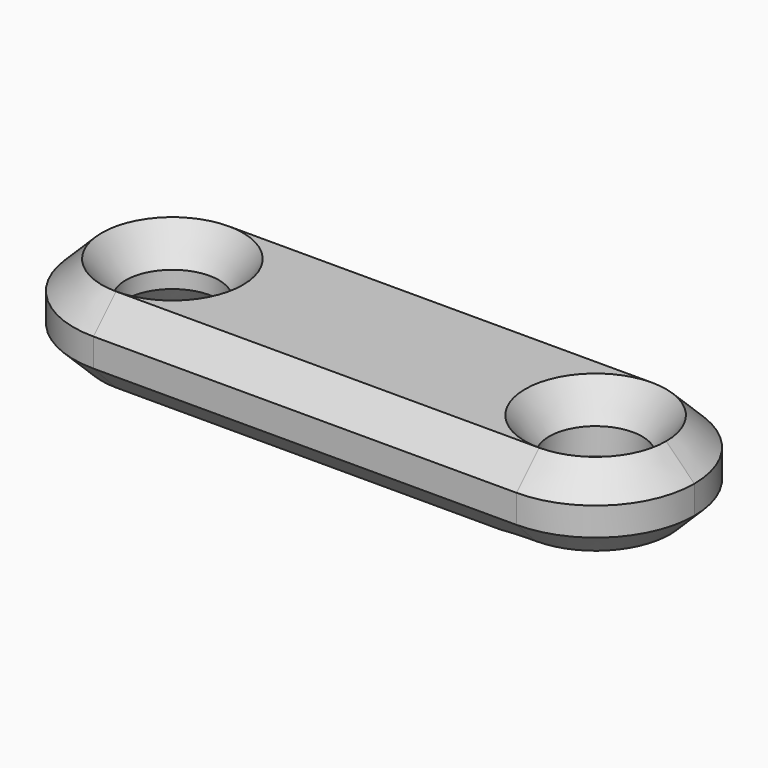
from build123d import *

# Parameters (mm, degrees)
F0_R     = 1.65
F1_DEPTH = 3
F2_SIZE  = 1


# Not quite as in the source:
# - a fillet or chamfer that OpenCascade refuses, or shapes differently, is made with other operations: its cross-section is extruded or revolved along the edge and cut away or added


with BuildPart() as f1:
    # F0 (on Top) → F1 (new body)
    with BuildSketch(Plane.XY):
        with BuildLine():
            ThreePointArc((-15, -3.5), (-12.5251262658, -2.4748737342), (-11.5, 0))
            ThreePointArc((-11.5, 0), (-12.5251262658, 2.4748737342), (-15, 3.5))
            ThreePointArc((-15, 3.5), (-18.5, 0), (-15, -3.5))
        make_face()
        with Locations((-15, 0)):
            Circle(F0_R, mode=Mode.SUBTRACT)
        with BuildLine():
            ThreePointArc((-15, 3.5), (-12.5251262658, 2.4748737342), (-11.5, 0))
            ThreePointArc((-11.5, 0), (-12.5251262658, -2.4748737342), (-15, -3.5))
            Line((-15, -3.5), (0, -3.5))
            ThreePointArc((0, -3.5), (-3.5, 0), (0, 3.5))
            Line((0, 3.5), (-15, 3.5))
        make_face()
        with BuildLine():
            ThreePointArc((3.5, 0), (2.4748737342, 2.4748737342), (0, 3.5))
            ThreePointArc((0, 3.5), (-3.5, 0), (0, -3.5))
            ThreePointArc((0, -3.5), (2.4748737342, -2.4748737342), (3.5, 0))
        make_face()
        Circle(F0_R, mode=Mode.SUBTRACT)
    extrude(amount=F1_DEPTH)

    # F2
    f2_edges = [f1.edges().sort_by_distance(p)[0] for p in [
        (-7.5, -3.5, 3),
        (-18.5, 0, 3),
        (3.5, 0, 3),
        (-7.5, 3.5, 3),
        (-7.5, -3.5, 0),
        (-18.5, 0, 0),
        (3.5, 0, 0),
        (-7.5, 3.5, 0),
    ]]
    chamfer(f2_edges, length=F2_SIZE)

    # F3: chamfer of 1.2 x 0.85 on 4 edges, made by hand

    # F3_s1 → F3_t2 (revolve, cut)
    with BuildSketch(Plane.XZ):
        Polygon((-12.5, 3), (-13.35, 1.8), (-13.35, 3), align=None)
    revolve(axis=Axis((-15, 0, 3), (0, 0, 1)), mode=Mode.SUBTRACT)

    # F3_s3 → F3_t4 (revolve, cut)
    with BuildSketch(Plane.XZ):
        Polygon((2.5, 3), (1.65, 1.8), (1.65, 3), align=None)
    revolve(axis=Axis((0, 0, 3), (0, 0, 1)), mode=Mode.SUBTRACT)

    # F3_s5 → F3_t6 (revolve, cut)
    with BuildSketch(Plane.XZ):
        Polygon((2.85, 0), (1.65, 0.85), (1.65, 0), align=None)
    revolve(axis=Axis((0, 0, 0), (0, 0, 1)), mode=Mode.SUBTRACT)

    # F3_s7 → F3_t8 (revolve, cut)
    with BuildSketch(Plane.XZ):
        Polygon((-12.5, 0), (-13.35, 1.2), (-13.35, 0), align=None)
    revolve(axis=Axis((-15, 0, 0), (0, 0, 1)), mode=Mode.SUBTRACT)


solid = f1.part
